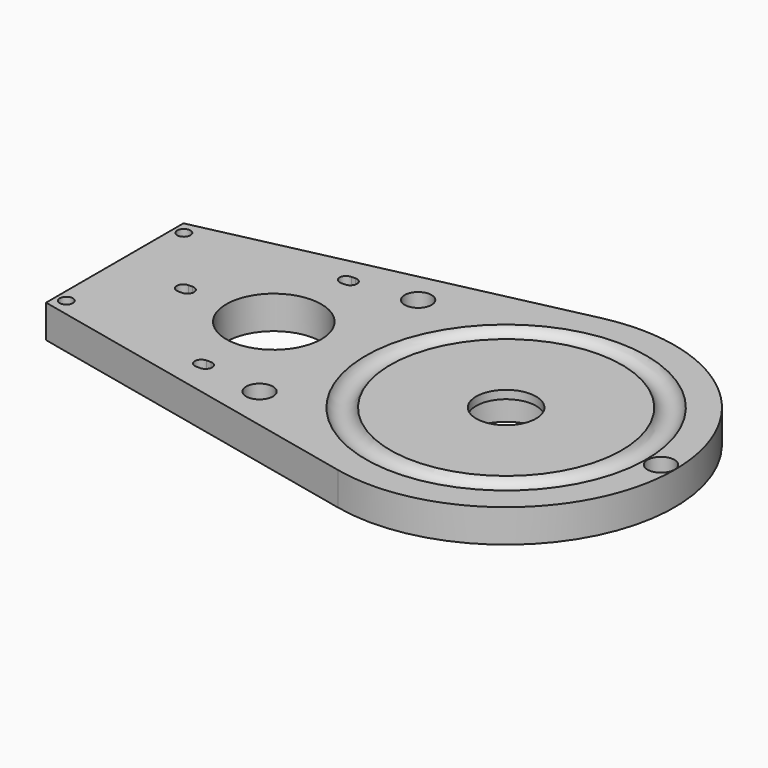
from build123d import *

# Parameters (mm, degrees)
F0_R            = 40.8
F1_DEPTH        = 8
F4_R            = 3.15
F6_W            = 4.8
F6_H            = 38.4
F7_DEPTH        = 8.001
F9_DEPTH        = 8
F10_R           = 11.5
F10_R_2         = 1.6
F11_DEPTH       = 8.001
F13_D           = 3.3
F13_CBORE_D     = 6.5
F13_CBORE_DEPTH = 6


# Not quite as in the source:
# - a feature names something its author has since deleted; it is built from what else it names


with BuildPart() as f1:
    # F0 (on Top) → F1 (new body)
    with BuildSketch(Plane.XY):
        Circle(F0_R)
    extrude(amount=F1_DEPTH)

    # F2 (on Right) → F3 (revolve, cut)
    with BuildSketch(Plane.YZ):
        Polygon((0, 8), (0, 0), (9.525, 0), (9.525, 6), (7.25, 6), (7.25, 8), align=None)
    revolve(axis=Axis((0, 0, 10.7360328796), (0, 0, 1)), mode=Mode.SUBTRACT)

    # F4 (on Right) → F5 (revolve, cut)
    with BuildSketch(Plane.YZ):
        with Locations((31, 9)):
            Circle(F4_R)
    revolve(axis=Axis((0, 0, 6.3867427816), (0, 0, 1)), mode=Mode.SUBTRACT)

    # F6 (on Top) → F7 (cut, through all)
    with BuildSketch(Plane.XY):
        with Locations((-38.4, 0)):
            Rectangle(F6_W, F6_H)
    extrude(amount=F7_DEPTH, mode=Mode.SUBTRACT)

    # F8 (on Top) → F9 (join, through all)
    with BuildSketch(Plane.XY):
        with BuildLine():
            Line((-94.75, 20.7850348986), (-94.75, -20.7850348986))
            Line((-94.75, -20.7850348986), (-8.8307362487, -39.8328770905))
            ThreePointArc((-8.8307362487, -39.8328770905), (-24.6754459414, -32.4924970969), (-36, -19.2))
            Line((-36, -19.2), (-36, 19.2))
            ThreePointArc((-36, 19.2), (-24.6754459414, 32.4924970969), (-8.8307362487, 39.8328770905))
            Line((-8.8307362487, 39.8328770905), (-94.75, 20.7850348986))
        make_face()
    extrude(amount=F9_DEPTH)

    # F10 (on face) → F11 (cut, through all)
    with BuildSketch(Plane.XY.offset(8)):
        with Locations((-56.25, 0)):
            Circle(F10_R)
        with Locations((-92.25, 17.7850348986)):
            Circle(F10_R_2)
        with Locations((-92.25, -17.7850348986)):
            Circle(F10_R_2)
        with BuildLine():
            Line((-55.2488153952, 23.5201616153), (-56.2488153952, 23.5201616153))
            ThreePointArc((-56.2488153952, 23.5201616153), (-57.848786069, 21.9104743704), (-56.2294412604, 20.3202789187))
            Line((-56.2294412604, 20.3202789187), (-55.2488153952, 20.3202789187))
            ThreePointArc((-55.2488153952, 20.3202789187), (-53.6488740469, 21.920220267), (-55.2488153952, 23.5201616153))
        make_face()
        with BuildLine():
            Line((-77.1680206657, 1.6075620275), (-78.1680206657, 1.6075620275))
            ThreePointArc((-78.1680206657, 1.6075620275), (-79.7679913396, 0.0172492724), (-78.1873948004, -1.5923206691))
            Line((-78.1873948004, -1.5923206691), (-77.1680206657, -1.5923206691))
            ThreePointArc((-77.1680206657, -1.5923206691), (-75.5680793174, 0.0076206792), (-77.1680206657, 1.6075620275))
        make_face()
        with BuildLine():
            Line((-55.2488164927, -20.3202952302), (-56.2488164927, -20.3202952302))
            ThreePointArc((-56.2488164927, -20.3202952302), (-57.8487871666, -21.9299824752), (-56.229442358, -23.5201779268))
            Line((-56.229442358, -23.5201779268), (-55.2488164927, -23.5201779268))
            ThreePointArc((-55.2488164927, -23.5201779268), (-53.6488751444, -21.9202365785), (-55.2488164927, -20.3202952302))
        make_face()
    extrude(amount=-F11_DEPTH, mode=Mode.SUBTRACT)

    # F13 (through all)
    with Locations(Plane.XY.offset(8)):
        with Locations((-40.5, 24), (-40.5, -24), (37.5, 0)):
            CounterBoreHole(F13_D / 2, F13_CBORE_D / 2, F13_CBORE_DEPTH)


solid = f1.part
